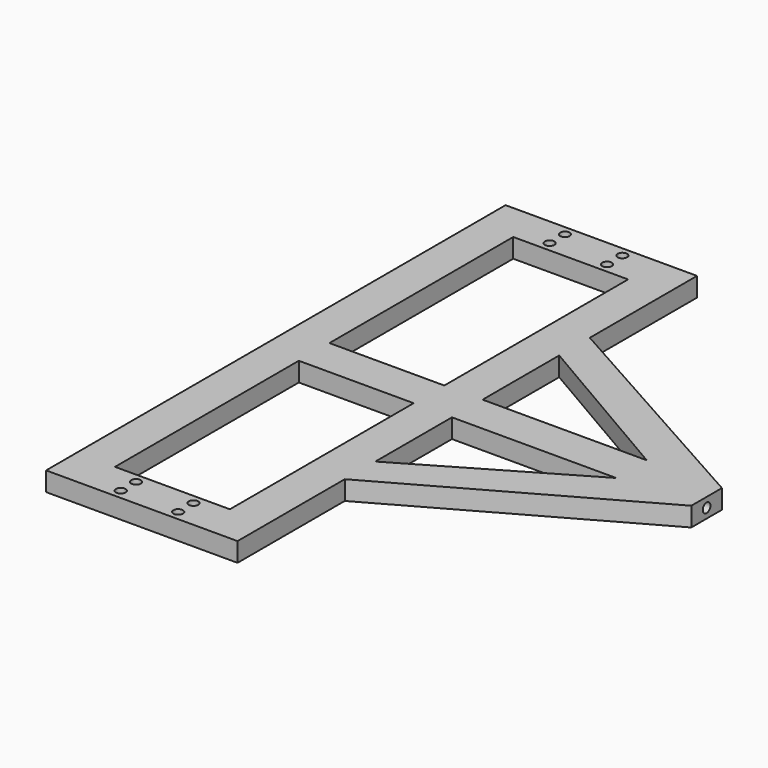
from build123d import *

# Parameters (mm, degrees)
F1_DEPTH = 20
F2_D     = 10
F3_D     = 10
F0_W     = 120
F0_H     = 40
F0_W_2   = 40
F4_DEPTH = 20
F6_D     = 10


# Not quite as in the source:
# - a feature names something its author has since deleted; it is built from what else it names


with BuildPart() as f1:
    # F0 (on Top) → F1 (new body)
    with BuildSketch(Plane.XY):
        Polygon((-359.5256319247, 349.3264111251), (-559.5256319247, 349.3264111251), (-559.5256319247, -250.6735888749), (-359.5256319247, -250.6735888749), (-359.5256319247, -110.6735888749), (-359.5256319247, -70.6735888749), (-359.5256319247, 29.3264111251), (-399.5256319247, 29.3264111251), (-399.5256319247, -210.6735888749), (-519.5256319247, -210.6735888749), (-519.5256319247, 29.3264111251), (-519.5256319247, 69.3264111251), (-519.5256319247, 309.3264111251), (-399.5256319247, 309.3264111251), (-399.5256319247, 69.3264111251), (-359.5256319247, 69.3264111251), (-359.5256319247, 169.3264111251), (-359.5256319247, 209.3264111251), align=None)
    extrude(amount=F1_DEPTH)

    # F2 (through all)
    with Locations(Plane(origin=(0, 0, 0), x_dir=(1, 0, 0), z_dir=(0, 0, -1))):
        with Locations((-489.5256319247, -339.3264111251), (-429.5256319247, -319.3264111251), (-489.5256319247, -319.3264111251), (-489.5256319247, 220.6735888749), (-489.5256319247, 240.6735888749), (-429.5256319247, 240.6735888749), (-429.5256319247, 220.6735888749)):
            Hole(F2_D / 2)

    # F3 (through all)
    with Locations(Plane(origin=(0, 0, 0), x_dir=(1, 0, 0), z_dir=(0, 0, -1))):
        with Locations((-429.5256319247, -339.3264111251)):
            Hole(F3_D / 2)

    # F0 (on Top) → F4 (join)
    with BuildSketch(Plane.XY):
        with Locations((-459.5256319247, 49.3264111251)):
            Rectangle(F0_W, F0_H)
        with Locations((-379.5256319247, 49.3264111251)):
            Rectangle(F0_W_2, F0_H)
        Polygon((-109.5256319247, 29.3264111251), (-109.5256319247, 69.3264111251), (-188.0447282525, 69.3264111251), (-359.5256319247, 69.3264111251), (-359.5256319247, 29.3264111251), (-188.0447282525, 29.3264111251), align=None)
        Polygon((-109.5256319247, 69.3264111251), (-359.5256319247, 209.3264111251), (-359.5256319247, 169.3264111251), (-188.0447282525, 69.3264111251), align=None)
        Polygon((-359.5256319247, -70.6735888749), (-359.5256319247, -110.6735888749), (-109.5256319247, 29.3264111251), (-188.0447282525, 29.3264111251), align=None)
    extrude(amount=F4_DEPTH)

    # F6 (through all)
    with Locations(Plane.YZ.offset(-109.5256319247)):
        with Locations((49.3264111251, 10)):
            Hole(F6_D / 2)


solid = f1.part
